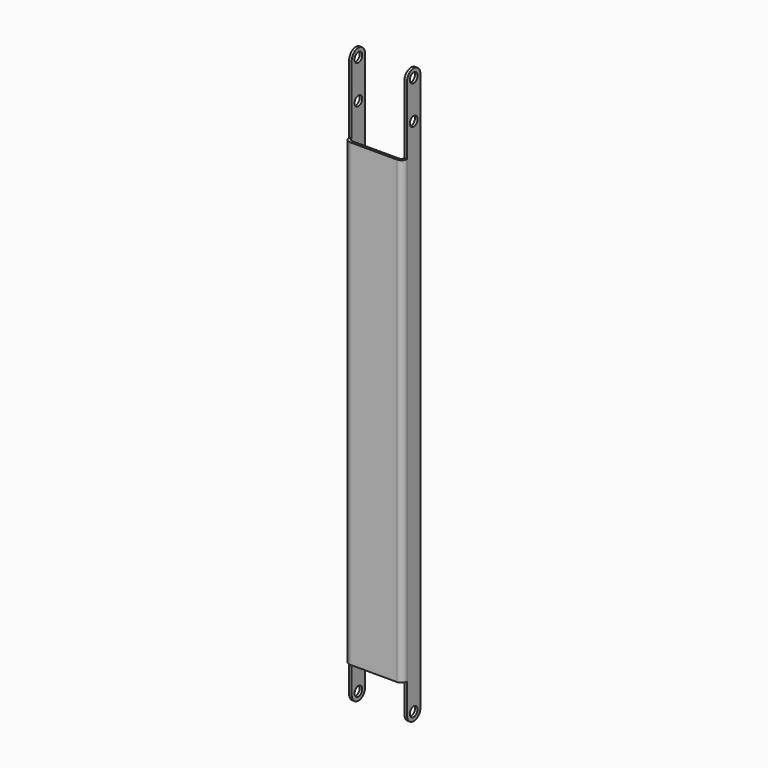
from build123d import *

# Parameters (mm, degrees)
F1_DEPTH = 304.8
F2_R     = 3.69316
F3_R     = 1.98374
F4_W     = 1.70942
F4_H     = 50.8
F4_H_2   = 25.4
F6_DEPTH = 11.1125
F7_R     = 5.55624
F8_R     = 3.175
F9_DEPTH = 38.36416


# Not quite as in the source:
# - a fillet or chamfer is up to 0.001 mm smaller than in the source, because OpenCascade refuses the exact size


with BuildPart() as f1:
    # F0 (on Top) → F1 (new body)
    with BuildSketch(Plane.XY):
        Polygon((0, 13.09624), (0, 0), (-34.94532, 0), (-34.94532, 13.09624), (-36.65474, 13.09624), (-36.65474, -1.70942), (1.70942, -1.70942), (1.70942, 13.09624), align=None)
    extrude(amount=F1_DEPTH)

    # F2
    f2_edges = [f1.edges().sort_by_distance(p)[0] for p in [
        (1.70942, -1.70942, 152.4),
        (-36.65474, -1.70942, 152.4),
    ]]
    fillet(f2_edges, radius=F2_R)

    # F3
    f3_edges = [f1.edges().sort_by_distance(p)[0] for p in [
        (0, 0, 152.4),
        (-34.94532, 0, 152.4),
    ]]
    fillet(f3_edges, radius=F3_R)

    # F4 (on face) → F6 (join, through all)
    with BuildSketch(Plane(origin=(0, 13.09624, 0), x_dir=(-1, 0, 0), z_dir=(0, 1, 0))):
        with Locations((35.80003, 330.2)):
            Rectangle(F4_W, F4_H)
        with Locations((-0.85471, 330.2)):
            Rectangle(F4_W, F4_H)
        with Locations((-0.85471, -12.7)):
            Rectangle(F4_W, F4_H_2)
        with Locations((35.80003, -12.7)):
            Rectangle(F4_W, F4_H_2)
    extrude(amount=-F6_DEPTH)

    # F7 (radius 5.55625 in the source; OpenCascade refuses exactly that, so slightly less here)
    f7_edges = [f1.edges().sort_by_distance(p)[0] for p in [
        (-35.80003, 13.09624, -25.4),
        (0.85471, 13.09624, -25.4),
        (0.85471, 13.09624, 355.6),
        (-35.80003, 13.09624, 355.6),
        (-35.80003, 1.98374, -25.4),
        (-35.80003, 1.98374, 355.6),
        (0.85471, 1.98374, 355.6),
        (0.85471, 1.98374, -25.4),
    ]]
    fillet(f7_edges, radius=F7_R)

    # F8 (on face) → F9 (cut, through all)
    with BuildSketch(Plane.YZ.offset(1.70942)):
        with Locations((7.53999, -19.84375)):
            Circle(F8_R)
        with Locations((7.53999, 350.04375)):
            Circle(F8_R)
        with Locations((7.53999, 324.64375)):
            Circle(F8_R)
    extrude(amount=-F9_DEPTH, mode=Mode.SUBTRACT)


solid = f1.part
